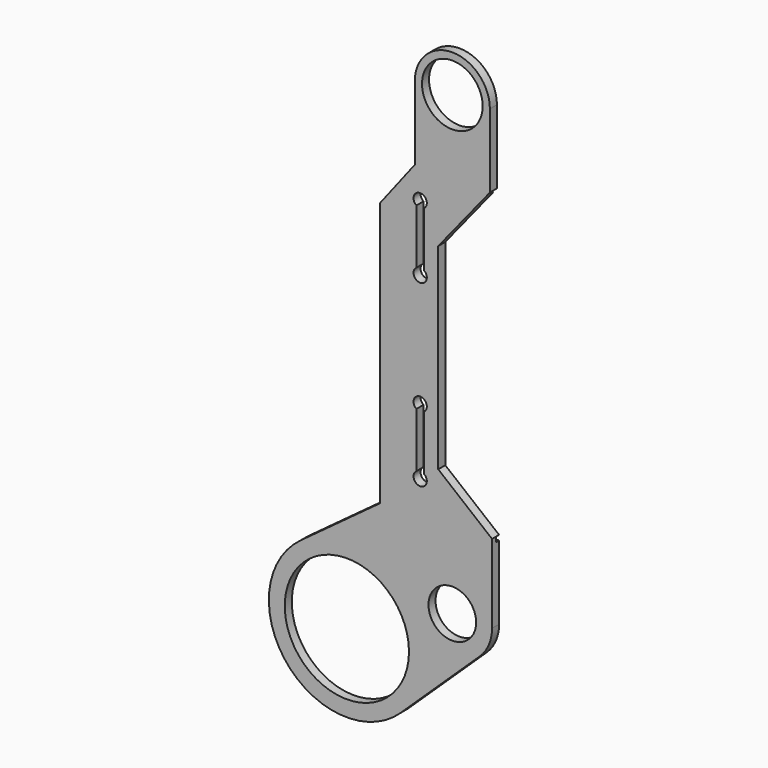
from build123d import *

# Parameters (mm, degrees)
F1_W     = 77.5
F1_H     = 3.475
F1_R     = 21
F1_R_2   = 43
F1_R_3   = 16.5
F2_DEPTH = 6.1
F3_DEPTH = 2.5


with BuildPart() as f2:
    # F1 (on Front) → F2 (new body)
    with BuildSketch(Plane.XZ):
        Polygon((100.5, -68.9009734364), (63.25, -38.5886058211), (63.25, 97.4589511752), (96.191884306, 138.2240265636), (44.3153656491, 138.2240265636), (23, 110.6333434582), (23, -68.9009734364), align=None)
        with BuildLine():
            Line((53.35, -27.8899289966), (53.35, -44.6062402442))
            ThreePointArc((53.35, -44.6062402442), (54.8193979899, -46.2562123774), (55.35, -48.4009734364))
            ThreePointArc((55.35, -48.4009734364), (48.605238941, -52.4703714262), (48.15, -44.6062402442))
            Line((48.15, -44.6062402442), (48.15, -27.8899289966))
            Line((48.15, -27.8899289966), (48.15, -25.6509734364))
            Line((48.15, -25.6509734364), (48.15, -23.4120178762))
            Line((48.15, -23.4120178762), (48.15, -6.6957066286))
            ThreePointArc((48.15, -6.6957066286), (48.605238941, 1.1684245535), (55.35, -2.9009734364))
            ThreePointArc((55.35, -2.9009734364), (54.8193979899, -5.0457344953), (53.35, -6.6957066286))
            Line((53.35, -6.6957066286), (53.35, -23.4120178762))
            Line((53.35, -23.4120178762), (53.35, -25.6509734364))
            Line((53.35, -25.6509734364), (53.35, -27.8899289966))
        make_face(mode=Mode.SUBTRACT)
        with BuildLine():
            Line((53.35, 98.1746025085), (53.35, 79.3937597558))
            ThreePointArc((53.35, 79.3937597558), (54.8193979899, 77.7437876226), (55.35, 75.5990265636))
            ThreePointArc((55.35, 75.5990265636), (48.605238941, 71.5296285738), (48.15, 79.3937597558))
            Line((48.15, 79.3937597558), (48.15, 98.1746025085))
            Line((48.15, 98.1746025085), (48.15, 98.3490265636))
            Line((48.15, 98.3490265636), (48.15, 98.5234506187))
            Line((48.15, 98.5234506187), (48.15, 117.3042933714))
            ThreePointArc((48.15, 117.3042933714), (48.605238941, 125.1684245535), (55.35, 121.0990265636))
            ThreePointArc((55.35, 121.0990265636), (54.8193979899, 118.9542655047), (53.35, 117.3042933714))
            Line((53.35, 117.3042933714), (53.35, 98.5234506187))
            Line((53.35, 98.5234506187), (53.35, 98.3490265636))
            Line((53.35, 98.3490265636), (53.35, 98.1746025085))
        make_face(mode=Mode.SUBTRACT)
        with Locations((61.75, -70.6384734364)):
            Rectangle(F1_W, F1_H)
        Polygon((44.3153656491, 138.2240265636), (96.191884306, 138.2240265636), (99, 141.6990265636), (47, 141.6990265636), align=None)
        with BuildLine():
            Line((100.5, -123.3759734364), (100.5, -72.3759734364))
            Line((100.5, -72.3759734364), (23, -72.3759734364))
            Line((23, -72.3759734364), (-32.0207315003, -112.894106478))
            ThreePointArc((-32.0207315003, -112.894106478), (-41.3632102296, -191.0903053398), (37.2681203413, -195.4539366155))
            Line((37.2681203413, -195.4539366155), (91.979135359, -143.2767880183))
            ThreePointArc((91.979135359, -143.2767880183), (98.2801920718, -134.200107989), (100.5, -123.3759734364))
        make_face()
        with BuildLine():
            ThreePointArc((34.2832199621, -192.3240812312), (-45.2648285285, -176.8381561958), (-4.3373528695, -106.8906928462))
            Line((-4.3373528695, -106.8906928462), (70.9764840916, -100.2894836995))
            ThreePointArc((70.9764840916, -100.2894836995), (94.11751185, -113.8297009562), (88.9942349798, -140.1469326341))
            Line((88.9942349798, -140.1469326341), (34.2832199621, -192.3240812312))
        make_face(mode=Mode.SUBTRACT)
        with BuildLine():
            Line((47, 141.6990265636), (99, 141.6990265636))
            Line((99, 141.6990265636), (99, 192.6990265636))
            ThreePointArc((99, 192.6990265636), (73, 218.6990265636), (47, 192.6990265636))
            Line((47, 192.6990265636), (47, 141.6990265636))
        make_face()
        with Locations((73, 192.6990265636)):
            Circle(F1_R, mode=Mode.SUBTRACT)
        with BuildLine():
            Line((70.9764840916, -100.2894836995), (-4.3373528695, -106.8906928462))
            ThreePointArc((-4.3373528695, -106.8906928462), (-45.2648285285, -176.8381561958), (34.2832199621, -192.3240812312))
            Line((34.2832199621, -192.3240812312), (88.9942349798, -140.1469326341))
            ThreePointArc((88.9942349798, -140.1469326341), (94.11751185, -113.8297009562), (70.9764840916, -100.2894836995))
        make_face()
        with BuildLine():
            Line((-4.016471706, -110.5516572381), (71.297365255, -103.9504480915))
            ThreePointArc((71.297365255, -103.9504480915), (90.7687801974, -115.3435111553), (86.4579323455, -137.4874601399))
            Line((86.4579323455, -137.4874601399), (31.7469173277, -189.6646087371))
            ThreePointArc((31.7469173277, -189.6646087371), (-41.9160968759, -175.3243459967), (-4.016471706, -110.5516572381))
        make_face(mode=Mode.SUBTRACT)
        with BuildLine():
            ThreePointArc((86.4579323455, -137.4874601399), (90.7687801974, -115.3435111553), (71.297365255, -103.9504480915))
            Line((71.297365255, -103.9504480915), (-4.016471706, -110.5516572381))
            ThreePointArc((-4.016471706, -110.5516572381), (-41.9160968759, -175.3243459967), (31.7469173277, -189.6646087371))
            Line((31.7469173277, -189.6646087371), (86.4579323455, -137.4874601399))
        make_face()
        with Locations((0, -156.3759734364)):
            Circle(F1_R_2, mode=Mode.SUBTRACT)
        with Locations((73, -123.3759734364)):
            Circle(F1_R_3, mode=Mode.SUBTRACT)
    extrude(amount=F2_DEPTH)

    # F1 (on Front) → F3 (cut)
    with BuildSketch(Plane.XZ):
        Polygon((44.3153656491, 138.2240265636), (96.191884306, 138.2240265636), (99, 141.6990265636), (47, 141.6990265636), align=None)
        with Locations((61.75, -70.6384734364)):
            Rectangle(F1_W, F1_H)
        with BuildLine():
            Line((70.9764840916, -100.2894836995), (-4.3373528695, -106.8906928462))
            ThreePointArc((-4.3373528695, -106.8906928462), (-45.2648285285, -176.8381561958), (34.2832199621, -192.3240812312))
            Line((34.2832199621, -192.3240812312), (88.9942349798, -140.1469326341))
            ThreePointArc((88.9942349798, -140.1469326341), (94.11751185, -113.8297009562), (70.9764840916, -100.2894836995))
        make_face()
        with BuildLine():
            Line((-4.016471706, -110.5516572381), (71.297365255, -103.9504480915))
            ThreePointArc((71.297365255, -103.9504480915), (90.7687801974, -115.3435111553), (86.4579323455, -137.4874601399))
            Line((86.4579323455, -137.4874601399), (31.7469173277, -189.6646087371))
            ThreePointArc((31.7469173277, -189.6646087371), (-41.9160968759, -175.3243459967), (-4.016471706, -110.5516572381))
        make_face(mode=Mode.SUBTRACT)
    extrude(amount=F3_DEPTH, mode=Mode.SUBTRACT)


solid = f2.part
